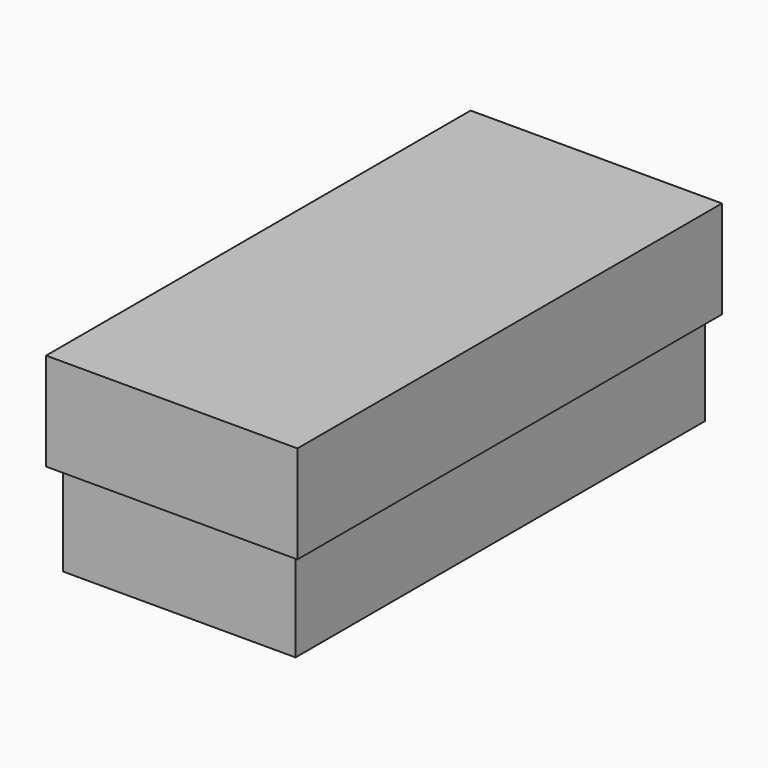
from build123d import *

# Parameters (mm, degrees)
F0_W     = 50
F0_H     = 110
F1_DEPTH = 40
F2_T     = -1
F3_W     = 54
F3_H     = 114
F3_W_2   = 50
F3_H_2   = 110
F3_W_3   = 48
F3_H_3   = 108
F4_DEPTH = 1
F5_DEPTH = 20
F6_W     = 48
F6_H     = 8
F7_DEPTH = 25
F9_DEPTH = 41.001


with BuildPart() as f1:
    # F0 (on Top) → F1 (new body)
    with BuildSketch(Plane.XY):
        with Locations((25, 55)):
            Rectangle(F0_W, F0_H)
    extrude(amount=F1_DEPTH)

    # F2
    f2_openings = [f1.faces().sort_by_distance(p)[0] for p in [
        (25, 55, 40),
    ]]
    offset(amount=F2_T, openings=f2_openings)


with BuildPart() as f4:
    # F3 (on face) → F4 (new body)
    with BuildSketch(Plane.XY.offset(40)):
        with Locations((25, 55)):
            Rectangle(F3_W, F3_H)
        with Locations((25, 55)):
            Rectangle(F3_W_2, F3_H_2, mode=Mode.SUBTRACT)
        with Locations((25, 55)):
            Rectangle(F3_W_2, F3_H_2)
        with Locations((25, 55)):
            Rectangle(F3_W_3, F3_H_3, mode=Mode.SUBTRACT)
        with Locations((25, 55)):
            Rectangle(F3_W_3, F3_H_3)
    extrude(amount=F4_DEPTH)

    # F3 (on face) → F5 (join)
    with BuildSketch(Plane.XY.offset(40)):
        with Locations((25, 55)):
            Rectangle(F3_W, F3_H)
        with Locations((25, 55)):
            Rectangle(F3_W_2, F3_H_2, mode=Mode.SUBTRACT)
    extrude(amount=-F5_DEPTH)


with BuildPart() as f7:
    # F6 (on face) → F7 (new body)
    with BuildSketch(Plane.XY.offset(1)):
        with Locations((25, 75)):
            Rectangle(F6_W, F6_H)
    extrude(amount=F7_DEPTH)

    # F8 (on face) → F9 (cut, through all)
    with BuildSketch(Plane.XZ.offset(-71)):
        with BuildLine():
            ThreePointArc((17.5, 26), (25, 18.5), (32.5, 26))
            Line((32.5, 26), (17.5, 26))
        make_face()
    extrude(amount=-F9_DEPTH, mode=Mode.SUBTRACT)


solid = Compound([f1.part, f4.part, f7.part])
